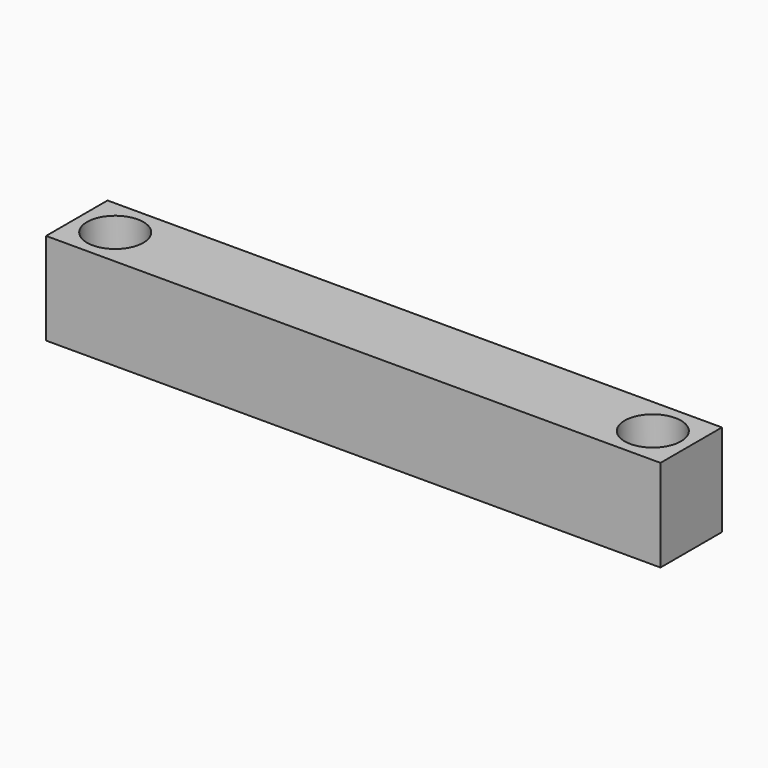
from build123d import *

# Parameters (mm, degrees)
F1_DEPTH         = 15
F2_W             = 74
F2_H             = 5
F3_DEPTH         = 15
F4_R             = 4.99999
F5_R             = 8
F8_D             = 7
F11_D            = 5
F11_DEPTH        = 20
F11_TIP          = 1.5021515476
F11_ON_F10_D     = 5
F11_ON_F10_DEPTH = 20
F11_ON_F10_TIP   = 1.5021515476
F12_W            = 105
F12_H            = 15
F12_W_2          = 15
F12_R            = 2.5
F13_DEPTH        = 18
F16_D            = 6.5
F16_CBORE_D      = 11
F16_CBORE_DEPTH  = 6.5


# Not quite as in the source:
# - a fillet or chamfer is up to 0.001 mm smaller than in the source, because OpenCascade refuses the exact size
# - a feature of the source that left no trace in its solid (it failed there, or was rolled back) is left out


with BuildPart() as f1:
    # F0 (on Front) → F1 (new body)
    with BuildSketch(Plane.XZ):
        Polygon((90, 0), (0, 0), (0, 61.5), (-15, 61.5), (-15, -15), (105, -15), (105, 61.5), (90, 61.5), align=None)
    extrude(amount=F1_DEPTH)

    # F2 (on face) → F3 (join, through all)
    with BuildSketch(Plane.XZ.offset(15)):
        with Locations((45, -17.5)):
            Rectangle(F2_W, F2_H)
    extrude(amount=-F3_DEPTH)

    # F4 (radius 5 in the source; OpenCascade refuses exactly that, so slightly less here)
    f4_edges = [f1.edges().sort_by_distance(p)[0] for p in [
        (0, -7.5, 0),
        (90, -7.5, 0),
        (8, -7.5, -15),
        (82, -7.5, -15),
    ]]
    fillet(f4_edges, radius=F4_R)

    # F5
    f5_edges = [f1.edges().sort_by_distance(p)[0] for p in [
        (-15, -7.5, -15),
        (105, -7.5, -15),
    ]]
    fillet(f5_edges, radius=F5_R)

    # F8 (through all)
    with Locations(Plane.XZ.offset(15)):
        with Locations((19.6, -10), (70.4, -10)):
            Hole(F8_D / 2)

    # F11
    with Locations(Plane.XY.offset(61.5)):
        with Locations((-7.5, -7.5)):
            Hole(F11_D / 2, depth=F11_DEPTH)
            with Locations((0, 0, -(F11_DEPTH + F11_TIP / 2))):  # 118° drill point
                Cone(0, F11_D / 2, F11_TIP, mode=Mode.SUBTRACT)

    # F11 on F10
    with Locations(Plane.XY.offset(61.5)):
        with Locations((97.5, -7.5)):
            Hole(F11_ON_F10_D / 2, depth=F11_ON_F10_DEPTH)
            with Locations((0, 0, -(F11_ON_F10_DEPTH + F11_ON_F10_TIP / 2))):  # 118° drill point
                Cone(0, F11_ON_F10_D / 2, F11_ON_F10_TIP, mode=Mode.SUBTRACT)


with BuildPart() as f13:
    # F12 (on face) → F13 (new body)
    with BuildSketch(Plane.XY.offset(61.5)):
        with Locations((52.5, -7.5)):
            Rectangle(F12_W, F12_H)
        with Locations((-7.5, -7.5)):
            Rectangle(F12_W_2, F12_H)
        with Locations((-7.5, -7.5)):
            Circle(F12_R, mode=Mode.SUBTRACT)
    extrude(amount=F13_DEPTH)

    # F16 (through all)
    with Locations(Plane.XY.offset(79.5)):
        with Locations((-7.5, -7.5), (97.5, -7.5)):
            CounterBoreHole(F16_D / 2, F16_CBORE_D / 2, F16_CBORE_DEPTH)


solid = f13.part
